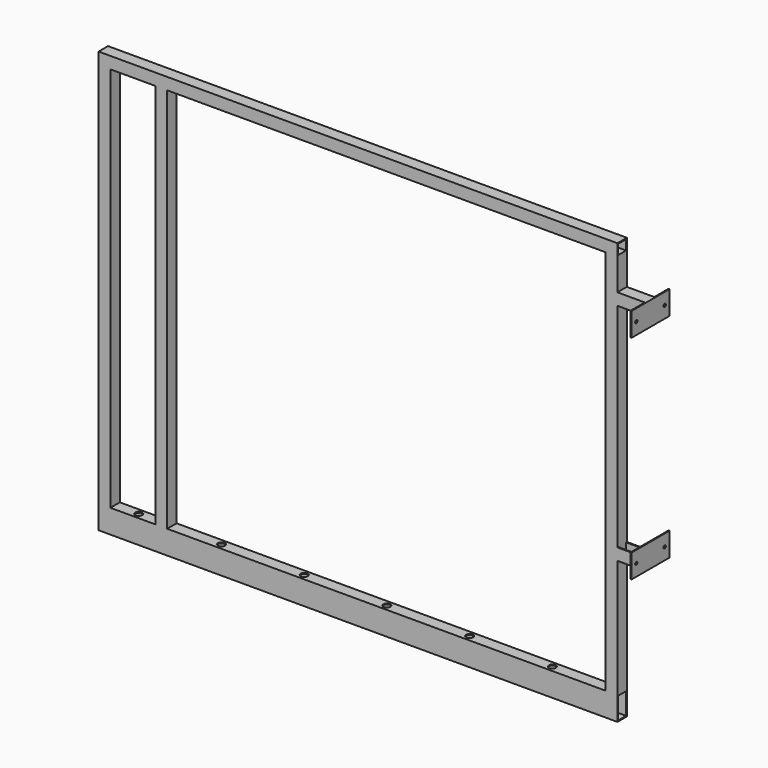
from build123d import *

# Parameters (mm, degrees)
F0_W      = 42
F0_H      = 42
F1_DEPTH  = 1633
F2_W      = 42
F2_H      = 92
F3_DEPTH  = 2195
F6_W      = 42
F6_H      = 42
F7_DEPTH  = 2195
F9_DEPTH  = 116
F10_W     = 200
F10_H     = 100
F10_R     = 6
F11_DEPTH = 4
F12_W     = 50
F12_H     = 50
F12_W_2   = 42
F12_H_2   = 42
F13_DEPTH = 1633
F14_R     = 7
F15_DEPTH = 125
F16_R     = 15
F16_R_2   = 7
F17_DEPTH = 5


# Not quite as in the source:
# - a feature names something its author has since deleted; it is built from what else it names


with BuildPart() as f1:
    # F0 (on Top) → F1 (new body)
    with BuildSketch(Plane.XY):
        Polygon((0, 4), (0, 0), (50, 0), (50, 50), (0, 50), (0, 46), align=None)
        with Locations((25, 25)):
            Rectangle(F0_W, F0_H, mode=Mode.SUBTRACT)
    extrude(amount=F1_DEPTH)


with BuildPart() as f3:
    # F2 (on face) → F3 (new body)
    with BuildSketch(Plane(origin=(0, 0, 0), x_dir=(0, -1, 0), z_dir=(-1, 0, 0))):
        Polygon((0, 0), (-50, 0), (-50, -4), (-50, -96), (-50, -100), (0, -100), align=None)
        with Locations((-25, -50)):
            Rectangle(F2_W, F2_H, mode=Mode.SUBTRACT)
    extrude(amount=-F3_DEPTH)

    # F5: F1 across plane
    add(f1.part.mirror(Plane.YZ.offset(1097.5)))


with BuildPart() as f1_1:
    add(f1.part)

    add(f3.part)  # F7 merges F3
    # F6 (on face) → F7 (join, through all)
    with BuildSketch(Plane(origin=(0, 0, 0), x_dir=(0, -1, 0), z_dir=(-1, 0, 0))):
        Polygon((-46, 1683), (-50, 1683), (-50, 1633), (0, 1633), (0, 1683), (-4, 1683), align=None)
        with Locations((-25, 1658)):
            Rectangle(F6_W, F6_H, mode=Mode.SUBTRACT)
    extrude(amount=-F7_DEPTH)

    # F8 (on face) → F9 (join)
    with BuildSketch(Plane.YZ.offset(2195)):
        Polygon((4, 550), (0, 550), (0, 500), (50, 500), (50, 550), (46, 550), (46, 504), (4, 504), align=None)
        Polygon((0, 1500), (0, 1450), (4, 1450), (4, 1496), (46, 1496), (46, 1450), (50, 1450), (50, 1500), align=None)
    extrude(amount=F9_DEPTH)

    # F10 (on face) → F11 (join)
    with BuildSketch(Plane.YZ.offset(2311)):
        with Locations((25, 1450)):
            Rectangle(F10_W, F10_H)
        with Locations((-50, 1450)):
            Circle(F10_R, mode=Mode.SUBTRACT)
        with Locations((100, 1450)):
            Circle(F10_R, mode=Mode.SUBTRACT)
        with Locations((25, 550)):
            Rectangle(F10_W, F10_H)
        with Locations((-50, 550)):
            Circle(F10_R, mode=Mode.SUBTRACT)
        with Locations((100, 550)):
            Circle(F10_R, mode=Mode.SUBTRACT)
    extrude(amount=F11_DEPTH)

    # F12 (on face) → F13 (join, through all)
    with BuildSketch(Plane.XY):
        with Locations((265, 25)):
            Rectangle(F12_W, F12_H)
        with Locations((265, 25)):
            Rectangle(F12_W_2, F12_H_2, mode=Mode.SUBTRACT)
    extrude(amount=F13_DEPTH)

    # F14 (on face) → F15 (cut)
    with BuildSketch(Plane(origin=(0, 0, -100), x_dir=(1, 0, 0), z_dir=(0, 0, -1))):
        with Locations((150, -25)):
            Circle(F14_R)
        with Locations((500, -25)):
            Circle(F14_R)
        with Locations((850, -25)):
            Circle(F14_R)
        with Locations((1200, -25)):
            Circle(F14_R)
        with Locations((1550, -25)):
            Circle(F14_R)
        with Locations((1900, -25)):
            Circle(F14_R)
        with Locations((2250, -25)):
            Circle(F14_R)
    extrude(amount=-F15_DEPTH, mode=Mode.SUBTRACT)

    # F16 (on face) → F17 (cut)
    with BuildSketch(Plane.XY):
        with Locations((500, 25)):
            Circle(F16_R)
        with Locations((500, 25)):
            Circle(F16_R_2, mode=Mode.SUBTRACT)
        with Locations((850, 25)):
            Circle(F16_R)
        with Locations((850, 25)):
            Circle(F16_R_2, mode=Mode.SUBTRACT)
        with Locations((1200, 25)):
            Circle(F16_R)
        with Locations((1200, 25)):
            Circle(F16_R_2, mode=Mode.SUBTRACT)
        with Locations((1550, 25)):
            Circle(F16_R)
        with Locations((1550, 25)):
            Circle(F16_R_2, mode=Mode.SUBTRACT)
        with Locations((1900, 25)):
            Circle(F16_R)
        with Locations((1900, 25)):
            Circle(F16_R_2, mode=Mode.SUBTRACT)
        with Locations((150, 25)):
            Circle(F16_R)
    extrude(amount=-F17_DEPTH, mode=Mode.SUBTRACT)


solid = f1_1.part
